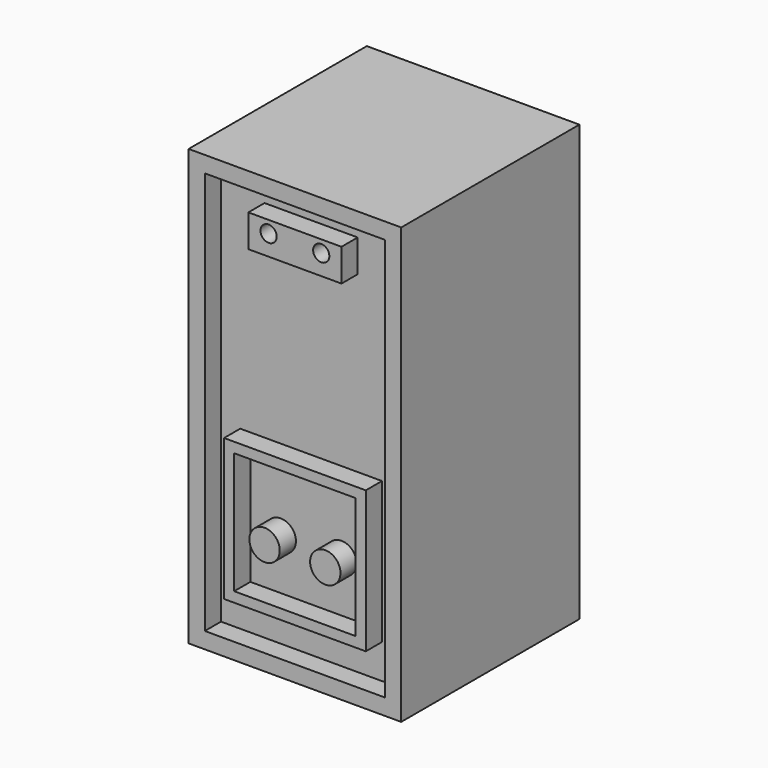
from build123d import *

# Parameters (mm, degrees)
F1_DEPTH  = 215
F2_SIZE   = 10
F3_R      = 20
F3_R_2    = 30
F4_DEPTH  = 8
F5_R      = 15
F5_R_2    = 25
F6_DEPTH  = 5
F7_R      = 4.99999
F8_R      = 15
F8_R_2    = 7.5
F9_DEPTH  = 5
F10_W     = 89
F10_H     = 199
F11_DEPTH = 10
F12_W     = 46
F12_H     = 16
F12_R     = 4
F13_DEPTH = 10
F14_W     = 70
F14_H     = 70
F14_W_2   = 60
F14_H_2   = 60
F14_R     = 7.5
F15_DEPTH = 10


# Not quite as in the source:
# - a fillet or chamfer is up to 0.001 mm smaller than in the source, because OpenCascade refuses the exact size


with BuildPart() as f1:
    # F0 (on Top) → F1 (new body)
    with BuildSketch(Plane.XY):
        Polygon((0, 110), (0, 0), (105, 0), (105, 110), (95, 120), (10, 120), align=None)
    extrude(amount=F1_DEPTH)

    # F2
    f2_edges = [f1.edges().sort_by_distance(p)[0] for p in [
        (52.5, 120, 215),
        (52.5, 120, 0),
    ]]
    chamfer(f2_edges, length=F2_SIZE)

    # F3 (on face) → F4 (cut)
    with BuildSketch(Plane(origin=(0, 120, 0), x_dir=(-1, 0, 0), z_dir=(0, 1, 0))):
        with Locations((-52.5, 150)):
            Circle(F3_R)
        with Locations((-52.5, 70)):
            Circle(F3_R_2)
    extrude(amount=-F4_DEPTH, mode=Mode.SUBTRACT)

    # F5 (on face) → F6 (join)
    with BuildSketch(Plane(origin=(0, 112, 0), x_dir=(-1, 0, 0), z_dir=(0, 1, 0))):
        with Locations((-52.5, 150)):
            Circle(F5_R)
        with Locations((-52.5, 70)):
            Circle(F5_R_2)
    extrude(amount=F6_DEPTH)

    # F7 (radius 5 in the source; OpenCascade refuses exactly that, so slightly less here)
    f7_edges = [f1.edges().sort_by_distance(p)[0] for p in [
        (77.5, 117, 70),
        (67.5, 117, 150),
    ]]
    fillet(f7_edges, radius=F7_R)

    # F8 (on face) → F9 (cut)
    with BuildSketch(Plane(origin=(0, 117, 0), x_dir=(-1, 0, 0), z_dir=(0, 1, 0))):
        with Locations((-52.5, 70)):
            Circle(F8_R)
        with Locations((-52.5, 70)):
            Circle(F8_R_2, mode=Mode.SUBTRACT)
    extrude(amount=-F9_DEPTH, mode=Mode.SUBTRACT)

    # F10 (on face) → F11 (cut)
    with BuildSketch(Plane.XZ):
        with Locations((52.5, 107.5)):
            Rectangle(F10_W, F10_H)
    extrude(amount=-F11_DEPTH, mode=Mode.SUBTRACT)

    # F12 (on face) → F13 (join)
    with BuildSketch(Plane.XZ.offset(-10)):
        with Locations((52.5, 189)):
            Rectangle(F12_W, F12_H)
        with Locations((39.5, 191)):
            Circle(F12_R, mode=Mode.SUBTRACT)
        with Locations((65.5, 191)):
            Circle(F12_R, mode=Mode.SUBTRACT)
    extrude(amount=F13_DEPTH)

    # F14 (on face) → F15 (join)
    with BuildSketch(Plane.XZ.offset(-10)):
        with Locations((52.5, 60)):
            Rectangle(F14_W, F14_H)
        with Locations((52.5, 60)):
            Rectangle(F14_W_2, F14_H_2, mode=Mode.SUBTRACT)
        with Locations((67.5, 55)):
            Circle(F14_R)
        with Locations((37.5, 55)):
            Circle(F14_R)
    extrude(amount=F15_DEPTH)


solid = f1.part
